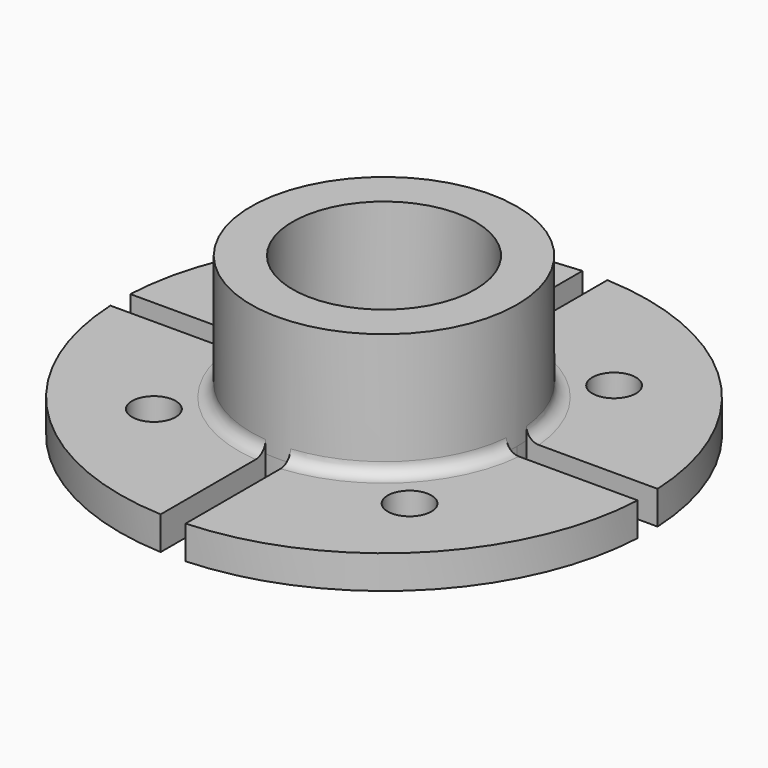
from build123d import *

# Parameters (mm, degrees)
F0_R         = 5.25
F1_DEPTH     = 8
F2_R         = 32
F2_R_2       = 22
F3_DEPTH     = 30
F4_T4_ANGLE  = 106.1070017135
F4_T9_ANGLE  = 106.1070017135
F4_T15_ANGLE = 106.1070017135
F4_T20_ANGLE = 106.1070017135
F4_T25_ANGLE = 106.1070017135
F4_T31_ANGLE = 106.1070017135
F4_T36_ANGLE = 106.1070017135
F4_T41_ANGLE = 106.1070017135
F4_T47_ANGLE = 106.1070017135
F4_T52_ANGLE = 106.1070017135
F4_T57_ANGLE = 106.1070017135
F4_T63_ANGLE = 106.1070017135
F5_R         = 5
F6_DEPTH     = 19.3


# Not quite as in the source:
# - a fillet or chamfer that OpenCascade refuses, or shapes differently, is made with other operations: its cross-section is extruded or revolved along the edge and cut away or added


with BuildPart() as f1:
    # F0 (on Top) → F1 (new body)
    with BuildSketch(Plane.XY):
        with BuildLine():
            ThreePointArc((3, 31.8590646441), (22.627416998, 22.627416998), (31.8590646441, 3))
            Line((31.8590646441, 3), (63.4290942707, 3))
            ThreePointArc((63.4290942707, 3), (44.9012806053, 44.9012806053), (3, 63.4290942707))
            Line((3, 63.4290942707), (3, 31.8590646441))
        make_face()
        with Locations((30.7591449816, 30.7591449816)):
            Circle(F0_R, mode=Mode.SUBTRACT)
        with BuildLine():
            ThreePointArc((-31.8590646441, 3), (-22.627416998, 22.627416998), (-3, 31.8590646441))
            Line((-3, 31.8590646441), (-3, 63.4290942707))
            ThreePointArc((-3, 63.4290942707), (-44.9012806053, 44.9012806053), (-63.4290942707, 3))
            Line((-63.4290942707, 3), (-31.8590646441, 3))
        make_face()
        with Locations((-30.7591449816, 30.7591449816)):
            Circle(F0_R, mode=Mode.SUBTRACT)
        with BuildLine():
            Line((-3, -63.4290942707), (-3, -31.8590646441))
            ThreePointArc((-3, -31.8590646441), (-22.627416998, -22.627416998), (-31.8590646441, -3))
            Line((-31.8590646441, -3), (-63.4290942707, -3))
            ThreePointArc((-63.4290942707, -3), (-44.9012806053, -44.9012806053), (-3, -63.4290942707))
        make_face()
        with Locations((-30.7591449816, -30.7591449816)):
            Circle(F0_R, mode=Mode.SUBTRACT)
        with BuildLine():
            Line((63.4290942707, -3), (31.8590646441, -3))
            ThreePointArc((31.8590646441, -3), (22.627416998, -22.627416998), (3, -31.8590646441))
            Line((3, -31.8590646441), (3, -63.4290942707))
            ThreePointArc((3, -63.4290942707), (44.9012806053, -44.9012806053), (63.4290942707, -3))
        make_face()
        with Locations((30.7591449816, -30.7591449816)):
            Circle(F0_R, mode=Mode.SUBTRACT)
        with BuildLine():
            ThreePointArc((31.8590646441, -3), (31.9647467424, -1.501654319), (32, 0))
            ThreePointArc((32, 0), (31.9647467424, 1.501654319), (31.8590646441, 3))
            ThreePointArc((31.8590646441, 3), (22.627416998, 22.627416998), (3, 31.8590646441))
            ThreePointArc((3, 31.8590646441), (0, 32), (-3, 31.8590646441))
            ThreePointArc((-3, 31.8590646441), (-22.627416998, 22.627416998), (-31.8590646441, 3))
            ThreePointArc((-31.8590646441, 3), (-32, 0), (-31.8590646441, -3))
            ThreePointArc((-31.8590646441, -3), (-22.627416998, -22.627416998), (-3, -31.8590646441))
            ThreePointArc((-3, -31.8590646441), (0, -32), (3, -31.8590646441))
            ThreePointArc((3, -31.8590646441), (22.627416998, -22.627416998), (31.8590646441, -3))
        make_face()
    extrude(amount=F1_DEPTH)

    # F2 (on face) → F3 (join)
    with BuildSketch(Plane.XY.offset(8)):
        Circle(F2_R)
        Circle(F2_R_2, mode=Mode.SUBTRACT)
    extrude(amount=F3_DEPTH)

    # F4: fillet of radius 3 on 6 edges, made by hand


with BuildPart() as f4_tool2:
    # F4_s3 → F4_t4 (revolve)
    with BuildSketch(Plane(origin=(0, 0, 0), x_dir=(0, 0, 1), z_dir=(-0.1400977189, -0.9901376819, 0))):
        with BuildLine():
            ThreePointArc((11, -32), (8.8786796564, -32.8786796564), (8, -35))
            Line((8, -35), (8, -32))
            Line((8, -32), (11, -32))
        make_face()
    revolve(axis=Axis((0, 0, 8), (0, 0, 1)), revolution_arc=F4_T4_ANGLE)

    split(bisect_by=Plane.XZ.offset(3), keep=Keep.TOP)


with BuildPart() as f1_1:
    add(f1.part)

    # F4_t1: union F4_tool2
    add(f4_tool2.part)


with BuildPart() as f4_tool7:
    # F4_s8 → F4_t9 (revolve)
    with BuildSketch(Plane(origin=(0, 0, 0), x_dir=(0, 0, 1), z_dir=(-0.1400977189, -0.9901376819, 0))):
        with BuildLine():
            ThreePointArc((11, -32), (8.8786796564, -32.8786796564), (8, -35))
            Line((8, -35), (8, -32))
            Line((8, -32), (11, -32))
        make_face()
    revolve(axis=Axis((0, 0, 8), (0, 0, 1)), revolution_arc=F4_T9_ANGLE)

    split(bisect_by=Plane.YZ.offset(3), keep=Keep.TOP)

    split(bisect_by=Plane.XZ.offset(-3), keep=Keep.BOTTOM)


with BuildPart() as f1_2:
    add(f1_1.part)

    # F4_t6: union F4_tool7
    add(f4_tool7.part)


with BuildPart() as f4_tool13:
    # F4_s14 → F4_t15 (revolve)
    with BuildSketch(Plane(origin=(0, 0, 0), x_dir=(0, 0, 1), z_dir=(-0.1400977189, -0.9901376819, 0))):
        with BuildLine():
            ThreePointArc((11, -32), (8.8786796564, -32.8786796564), (8, -35))
            Line((8, -35), (8, -32))
            Line((8, -32), (11, -32))
        make_face()
    revolve(axis=Axis((0, 0, 8), (0, 0, 1)), revolution_arc=F4_T15_ANGLE)

    split(bisect_by=Plane.YZ.offset(-3), keep=Keep.BOTTOM)


with BuildPart() as f1_3:
    add(f1_2.part)

    # F4_t12: union F4_tool13
    add(f4_tool13.part)


with BuildPart() as f4_tool18:
    # F4_s19 → F4_t20 (revolve)
    with BuildSketch(Plane(origin=(0, 0, 0), x_dir=(0, 0, 1), z_dir=(-0.9901376819, 0.1400977189, 0))):
        with BuildLine():
            ThreePointArc((11, -32), (8.8786796564, -32.8786796564), (8, -35))
            Line((8, -35), (8, -32))
            Line((8, -32), (11, -32))
        make_face()
    revolve(axis=Axis((0, 0, 8), (0, 0, 1)), revolution_arc=F4_T20_ANGLE)

    split(bisect_by=Plane.YZ.offset(-3), keep=Keep.BOTTOM)


with BuildPart() as f1_4:
    add(f1_3.part)

    # F4_t17: union F4_tool18
    add(f4_tool18.part)


with BuildPart() as f4_tool23:
    # F4_s24 → F4_t25 (revolve)
    with BuildSketch(Plane(origin=(0, 0, 0), x_dir=(0, 0, 1), z_dir=(-0.9901376819, 0.1400977189, 0))):
        with BuildLine():
            ThreePointArc((11, -32), (8.8786796564, -32.8786796564), (8, -35))
            Line((8, -35), (8, -32))
            Line((8, -32), (11, -32))
        make_face()
    revolve(axis=Axis((0, 0, 8), (0, 0, 1)), revolution_arc=F4_T25_ANGLE)

    split(bisect_by=Plane.XZ.offset(3), keep=Keep.TOP)

    split(bisect_by=Plane.YZ.offset(3), keep=Keep.TOP)


with BuildPart() as f1_5:
    add(f1_4.part)

    # F4_t22: union F4_tool23
    add(f4_tool23.part)


with BuildPart() as f4_tool29:
    # F4_s30 → F4_t31 (revolve)
    with BuildSketch(Plane(origin=(0, 0, 0), x_dir=(0, 0, 1), z_dir=(-0.9901376819, 0.1400977189, 0))):
        with BuildLine():
            ThreePointArc((11, -32), (8.8786796564, -32.8786796564), (8, -35))
            Line((8, -35), (8, -32))
            Line((8, -32), (11, -32))
        make_face()
    revolve(axis=Axis((0, 0, 8), (0, 0, 1)), revolution_arc=F4_T31_ANGLE)

    split(bisect_by=Plane.XZ.offset(-3), keep=Keep.BOTTOM)


with BuildPart() as f1_6:
    add(f1_5.part)

    # F4_t28: union F4_tool29
    add(f4_tool29.part)


with BuildPart() as f4_tool34:
    # F4_s35 → F4_t36 (revolve)
    with BuildSketch(Plane(origin=(0, 0, 0), x_dir=(0, 0, 1), z_dir=(0.1400977189, 0.9901376819, 0))):
        with BuildLine():
            ThreePointArc((11, -32), (8.8786796564, -32.8786796564), (8, -35))
            Line((8, -35), (8, -32))
            Line((8, -32), (11, -32))
        make_face()
    revolve(axis=Axis((0, 0, 8), (0, 0, 1)), revolution_arc=F4_T36_ANGLE)

    split(bisect_by=Plane.XZ.offset(-3), keep=Keep.BOTTOM)


with BuildPart() as f1_7:
    add(f1_6.part)

    # F4_t33: union F4_tool34
    add(f4_tool34.part)


with BuildPart() as f4_tool39:
    # F4_s40 → F4_t41 (revolve)
    with BuildSketch(Plane(origin=(0, 0, 0), x_dir=(0, 0, 1), z_dir=(0.1400977189, 0.9901376819, 0))):
        with BuildLine():
            ThreePointArc((11, -32), (8.8786796564, -32.8786796564), (8, -35))
            Line((8, -35), (8, -32))
            Line((8, -32), (11, -32))
        make_face()
    revolve(axis=Axis((0, 0, 8), (0, 0, 1)), revolution_arc=F4_T41_ANGLE)

    split(bisect_by=Plane.XZ.offset(3), keep=Keep.TOP)

    split(bisect_by=Plane.YZ.offset(-3), keep=Keep.BOTTOM)


with BuildPart() as f1_8:
    add(f1_7.part)

    # F4_t38: union F4_tool39
    add(f4_tool39.part)


with BuildPart() as f4_tool45:
    # F4_s46 → F4_t47 (revolve)
    with BuildSketch(Plane(origin=(0, 0, 0), x_dir=(0, 0, 1), z_dir=(0.1400977189, 0.9901376819, 0))):
        with BuildLine():
            ThreePointArc((11, -32), (8.8786796564, -32.8786796564), (8, -35))
            Line((8, -35), (8, -32))
            Line((8, -32), (11, -32))
        make_face()
    revolve(axis=Axis((0, 0, 8), (0, 0, 1)), revolution_arc=F4_T47_ANGLE)

    split(bisect_by=Plane.YZ.offset(3), keep=Keep.TOP)


with BuildPart() as f1_9:
    add(f1_8.part)

    # F4_t44: union F4_tool45
    add(f4_tool45.part)


with BuildPart() as f4_tool50:
    # F4_s51 → F4_t52 (revolve)
    with BuildSketch(Plane(origin=(0, 0, 0), x_dir=(0, 0, 1), z_dir=(0.9901376819, -0.1400977189, 0))):
        with BuildLine():
            ThreePointArc((11, -32), (8.8786796564, -32.8786796564), (8, -35))
            Line((8, -35), (8, -32))
            Line((8, -32), (11, -32))
        make_face()
    revolve(axis=Axis((0, 0, 8), (0, 0, 1)), revolution_arc=F4_T52_ANGLE)

    split(bisect_by=Plane.YZ.offset(3), keep=Keep.TOP)


with BuildPart() as f1_10:
    add(f1_9.part)

    # F4_t49: union F4_tool50
    add(f4_tool50.part)


with BuildPart() as f4_tool55:
    # F4_s56 → F4_t57 (revolve)
    with BuildSketch(Plane(origin=(0, 0, 0), x_dir=(0, 0, 1), z_dir=(0.9901376819, -0.1400977189, 0))):
        with BuildLine():
            ThreePointArc((11, -32), (8.8786796564, -32.8786796564), (8, -35))
            Line((8, -35), (8, -32))
            Line((8, -32), (11, -32))
        make_face()
    revolve(axis=Axis((0, 0, 8), (0, 0, 1)), revolution_arc=F4_T57_ANGLE)

    split(bisect_by=Plane.XZ.offset(-3), keep=Keep.BOTTOM)

    split(bisect_by=Plane.YZ.offset(-3), keep=Keep.BOTTOM)


with BuildPart() as f1_11:
    add(f1_10.part)

    # F4_t54: union F4_tool55
    add(f4_tool55.part)


with BuildPart() as f4_tool61:
    # F4_s62 → F4_t63 (revolve)
    with BuildSketch(Plane(origin=(0, 0, 0), x_dir=(0, 0, 1), z_dir=(0.9901376819, -0.1400977189, 0))):
        with BuildLine():
            ThreePointArc((11, -32), (8.8786796564, -32.8786796564), (8, -35))
            Line((8, -35), (8, -32))
            Line((8, -32), (11, -32))
        make_face()
    revolve(axis=Axis((0, 0, 8), (0, 0, 1)), revolution_arc=F4_T63_ANGLE)

    split(bisect_by=Plane.XZ.offset(3), keep=Keep.TOP)


with BuildPart() as f1_12:
    add(f1_11.part)

    # F4_t60: union F4_tool61
    add(f4_tool61.part)

    # F5 (on face) → F6 (cut)
    with BuildSketch(Plane.XY.offset(8)):
        Circle(F5_R)
    extrude(amount=-F6_DEPTH, mode=Mode.SUBTRACT)


solid = f1_12.part
